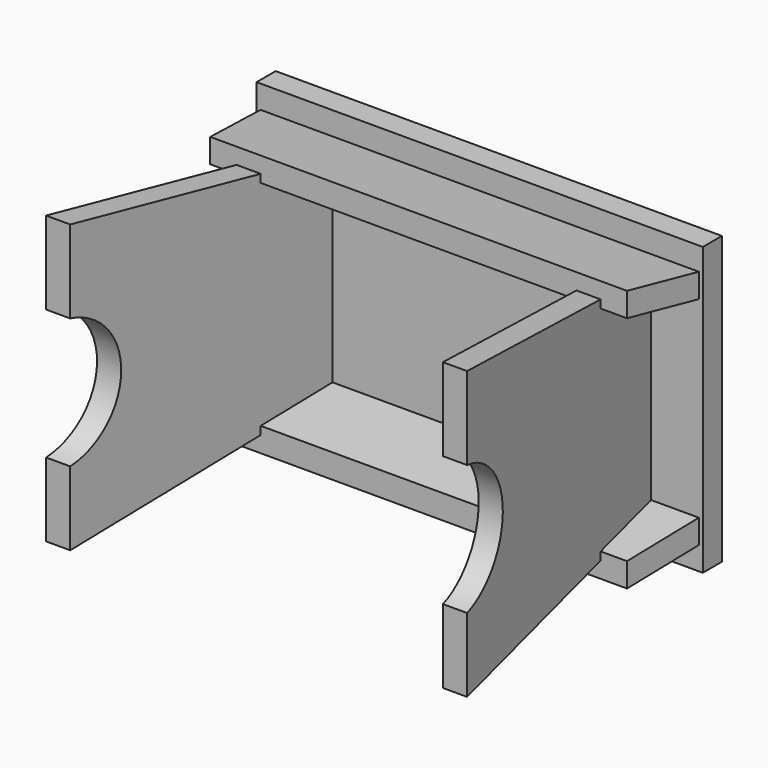
from build123d import *

# Parameters (mm, degrees)
F1_DEPTH      = 114.3
F2_DEPTH      = 114.3
F2_DEPTH_BACK = 114.3
F3_DEPTH      = 114.3
F3_DEPTH_BACK = 114.3
F5_DEPTH      = 177.801
F5_DEPTH_BACK = 177.801
F7_DEPTH      = 177.8
F7_DEPTH_BACK = 177.8
F8_DEPTH      = 114.3
F8_DEPTH_BACK = 114.3


# Not quite as in the source:
# - an extrude ends at something that could not be found from the text; its depth is read off the source's solid


with BuildPart() as f1:
    # F0 (on Top) → F1 (new body, symmetric)
    with BuildSketch(Plane.XY):
        Polygon((-177.8, 0), (-177.8, -19.05), (-174.625, -19.05), (-136.5145635031, -19.05), (-117.2773482466, -19.05), (0, -19.05), (0, 0), align=None)
        Polygon((177.8, 0), (0, 0), (0, -19.05), (117.2773482466, -19.05), (136.5145635031, -19.05), (174.625, -19.05), (177.8, -19.05), align=None)
    extrude(amount=F1_DEPTH, both=True)


with BuildPart() as f2:
    # F0 (on Top) → F2 (new body, two sides)
    with BuildSketch(Plane.XY) as f2_sk:
        Polygon((136.5145635031, -19.05), (117.2773482466, -19.05), (125.8289445898, -79.8977696986), (145.0661598463, -79.8977696986), align=None)
        Polygon((145.0661598463, -79.8977696986), (125.8289445898, -79.8977696986), (148.5125487592, -241.3), (167.7497640157, -241.3), align=None)
    extrude(amount=-F2_DEPTH)
    extrude(f2_sk.sketch, amount=F2_DEPTH_BACK)


with BuildPart() as f3:
    # F0 (on Top) → F3 (new body, two sides)
    with BuildSketch(Plane.XY) as f3_sk:
        Polygon((-117.2773482466, -19.05), (-136.5145635031, -19.05), (-145.0661598463, -79.8977696986), (-125.8289445898, -79.8977696986), align=None)
        Polygon((-125.8289445898, -79.8977696986), (-145.0661598463, -79.8977696986), (-167.7497640157, -241.3), (-148.5125487592, -241.3), align=None)
    extrude(amount=F3_DEPTH)
    extrude(f3_sk.sketch, amount=-F3_DEPTH_BACK)


with BuildPart() as f5_tool:
    # F4 (on Right) → F5 (new body, two sides)
    with BuildSketch(Plane.YZ) as f5_sk:
        with BuildLine():
            Line((-241.3, 48.3545251191), (-241.3, -55.417560041))
            ThreePointArc((-241.3, -55.417560041), (-198.1072526182, -3.5315174609), (-241.3, 48.3545251191))
        make_face()
        Polygon((-241.3, -114.2999999998), (-19.05, -114.2999999998), (-19.05, -83.0647994877), align=None)
        Polygon((-241.3, 114.3000000004), (-19.05, 83.0647994877), (-19.05, 114.3000000004), align=None)
    extrude(amount=-F5_DEPTH)
    extrude(f5_sk.sketch, amount=F5_DEPTH_BACK)


with BuildPart() as f2_1:
    add(f2.part)

    # F5: cut by f5_tool
    add(f5_tool.part, mode=Mode.SUBTRACT)


with BuildPart() as f3_1:
    add(f3.part)

    # F5: cut by f5_tool
    add(f5_tool.part, mode=Mode.SUBTRACT)


with BuildPart() as f7:
    # F6 (on Right) → F7 (new body, two sides)
    with BuildSketch(Plane.YZ) as f7_sk:
        Polygon((-19.0500000004, -83.0647994877), (-19.0500000003, -76.6523944022), (-79.8977696986, -85.2039907455), (-79.8977696986, -91.616395831), align=None)
        Polygon((-19.0500000004, -95.8896096587), (-19.0500000004, -83.0647994877), (-79.8977696986, -91.616395831), (-79.8977696986, -104.4412060019), align=None)
    extrude(amount=F7_DEPTH)
    extrude(f7_sk.sketch, amount=-F7_DEPTH_BACK)


with BuildPart() as f7b:
    # F6 (on Right) → F7, piece 2 (new body, two sides)
    with BuildSketch(Plane.YZ) as f7_2_sk:
        Polygon((-19.0499999999, 76.6523944022), (-19.0499999999, 83.0647994877), (-79.8977696986, 91.616395831), (-79.8977696986, 85.2039907455), align=None)
        Polygon((-79.8977696986, 91.616395831), (-19.05, 83.0647994877), (-19.0499999999, 95.8896096587), (-79.8977696986, 104.4412060019), align=None)
    extrude(amount=F7_DEPTH)
    extrude(f7_2_sk.sketch, amount=-F7_DEPTH_BACK)


with BuildPart() as f8_tool:
    # F0 (on Top) → F8 (new body, two sides)
    with BuildSketch(Plane.XY) as f8_sk:
        Polygon((177.8, -79.8977696986), (177.8, -19.05), (174.625, -19.05), (166.0734036568, -79.8977696986), align=None)
        Polygon((-174.625, -19.05), (-177.8, -19.05), (-177.8, -79.8977696986), (-166.0734036568, -79.8977696986), align=None)
    extrude(amount=F8_DEPTH)
    extrude(f8_sk.sketch, amount=-F8_DEPTH_BACK)


with BuildPart() as f7_1:
    add(f7.part)

    # F8: cut by f8_tool
    add(f8_tool.part, mode=Mode.SUBTRACT)

    # F11: cut F2
    add(f2_1.part, mode=Mode.SUBTRACT)

    # F12: cut F3
    add(f3_1.part, mode=Mode.SUBTRACT)


with BuildPart() as f7b_1:
    add(f7b.part)

    # F8: cut by f8_tool
    add(f8_tool.part, mode=Mode.SUBTRACT)

    # F9: cut F3
    add(f3_1.part, mode=Mode.SUBTRACT)

    # F10: cut F2
    add(f2_1.part, mode=Mode.SUBTRACT)


solid = Compound([f1.part, f2_1.part, f3_1.part, f7_1.part, f7b_1.part])
